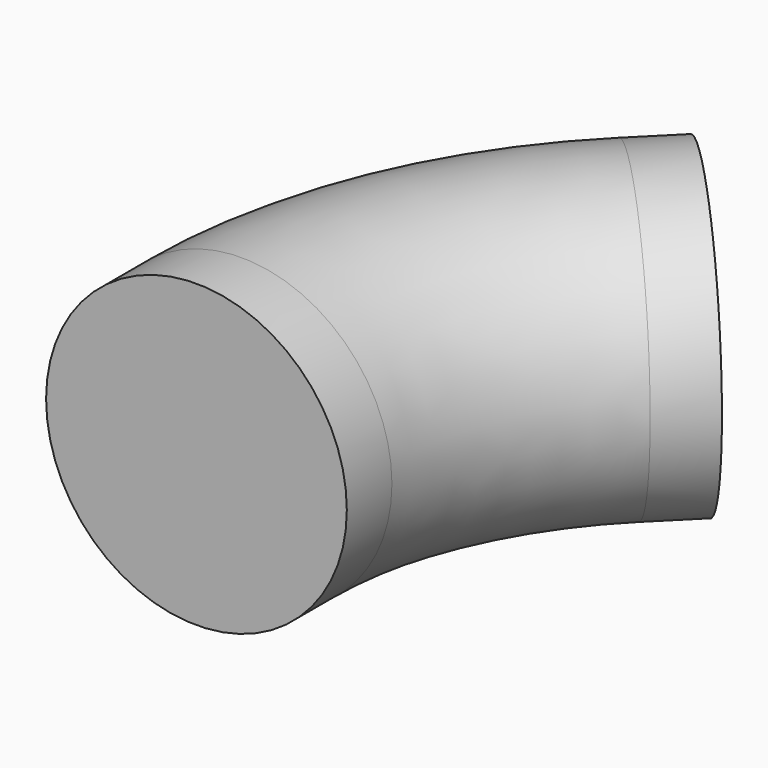
from build123d import *

# Parameters (mm, degrees)
F0_R     = 152.4
F3_DEPTH = 57.15
F4_DEPTH = 57.15


with BuildPart() as f2:
    # F2: sweep along a path in F1
    with BuildLine(Plane.XY) as f2_path:
        ThreePointArc((-323.2892203585, 323.2892203585), (-422.3977222642, 174.9628652773), (-457.2, 0))
    # F0 (on Front) → F2 (sweep)
    with BuildSketch(Plane.XZ):
        with Locations((-457.2, 0)):
            Circle(F0_R)
    sweep(path=f2_path.line)

    # F3 (add): a face of the model
    f3_faces = [f2.faces().sort_by_distance(p)[0] for p in [
        (-457.2, 0, 0),
    ]]
    extrude(f3_faces, amount=F3_DEPTH)

    # F4 (add): a face of the model
    f4_faces = [f2.faces().sort_by_distance(p)[0] for p in [
        (-323.2892203585, 323.2892203585, 0),
    ]]
    extrude(f4_faces, amount=F4_DEPTH)


solid = f2.part
